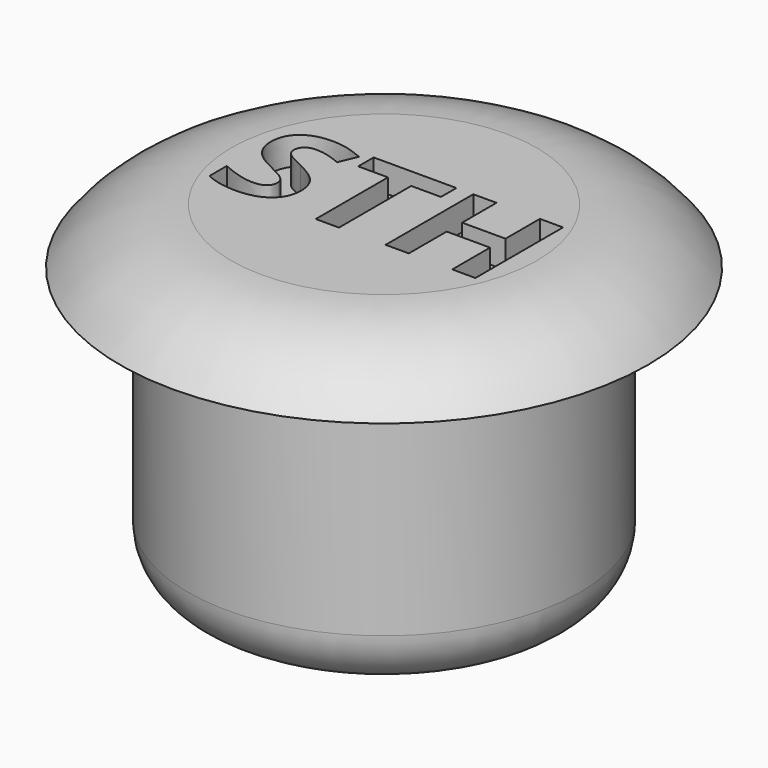
from build123d import *

# Parameters (mm, degrees)
F0_R         = 7.055
F1_DEPTH     = 10
F2_R         = 9.5
F2_R_2       = 7.055
F3_DEPTH     = 2
F5_R         = 2
F6_TEXT_SIZE = 5.5242722738
F7_DEPTH     = 1
F8_DEPTH     = 7


# Not quite as in the source:
# - a fillet or chamfer that OpenCascade refuses, or shapes differently, is made with other operations: its cross-section is extruded or revolved along the edge and cut away or added
# - Text() gives the source's letters only with a copy of the font that has no kerning and outlines rounded to 1/6400 em; it was checked with that copy


with BuildPart() as f1:
    # F0 (on Top) → F1 (new body)
    with BuildSketch(Plane.XY):
        Circle(F0_R)
    extrude(amount=F1_DEPTH)

    # F2 (on face) → F3 (join)
    with BuildSketch(Plane.XY.offset(10)):
        Circle(F2_R)
        Circle(F2_R_2, mode=Mode.SUBTRACT)
        Circle(F2_R_2)
    extrude(amount=F3_DEPTH)

    # F4: fillet of radius 5 on 1 edges, made by hand

    # F4_s1 → F4_t2 (revolve, cut)
    with BuildSketch(Plane.XZ):
        with BuildLine():
            ThreePointArc((9.5, 10), (7.7360679775, 11.472135955), (5.5, 12))
            Line((5.5, 12), (9.5, 12))
            Line((9.5, 12), (9.5, 10))
        make_face()
    revolve(axis=Axis((0, 0, 12), (0, 0, 1)), mode=Mode.SUBTRACT)

    # F5
    f5_edges = [f1.edges().sort_by_distance(p)[0] for p in [
        (-7.055, 0, 0),
    ]]
    fillet(f5_edges, radius=F5_R)

    # F6 (on face) → F7 (cut)
    with BuildSketch(Plane.XY.offset(12)):
        with Locations((-5.1620024988, -1.8983493362)):
            Text('STH', F6_TEXT_SIZE, font='Open Sans', font_style=FontStyle.BOLD, text_align=(TextAlign.LEFT, TextAlign.BOTTOM))
    extrude(amount=-F7_DEPTH, mode=Mode.SUBTRACT)

    # F8 (cut): a face of the model
    f8_faces = [f1.faces().sort_by_distance(p)[0] for p in [
        (0, 0, 0),
    ]]
    extrude(f8_faces, amount=-F8_DEPTH, mode=Mode.SUBTRACT)


solid = f1.part
